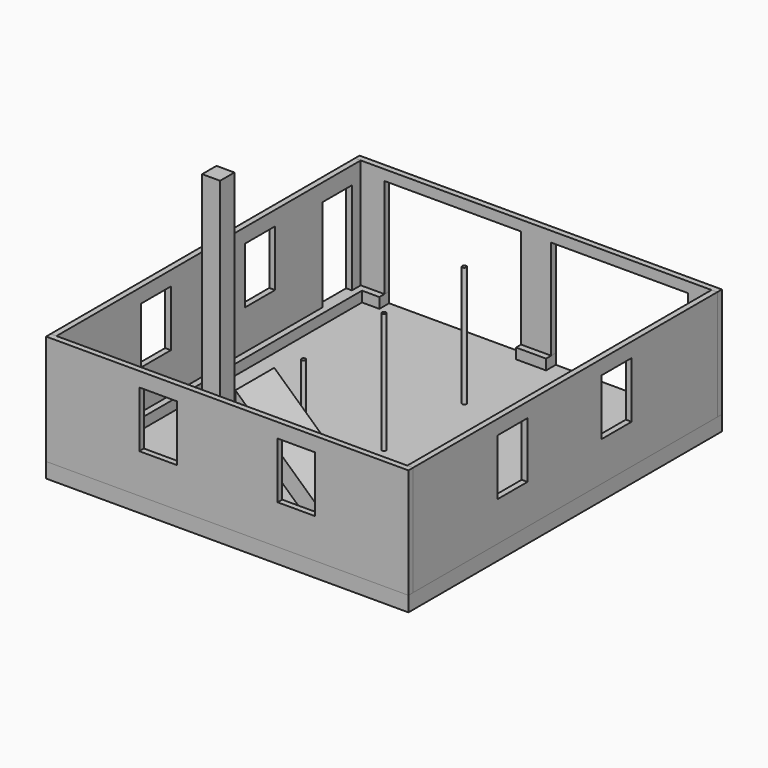
from build123d import *

# Parameters (mm, degrees)
F0_W      = 7950.2
F0_H      = 8597.9
F1_DEPTH  = 101.6
F2_W      = 660.4
F2_H      = 266.7
F3_DEPTH  = 228.6
F5_DEPTH  = 127
F6_W      = 7950.2
F6_H      = 2413
F6_W_2    = 825.5
F6_H_2    = 1231.9
F7_DEPTH  = 127
F8_W      = 825.5
F8_H      = 1231.9
F9_DEPTH  = 127
F10_W     = 8343.9
F10_H     = 2413
F11_DEPTH = 127
F12_DEPTH = 7950.2
F13_W     = 393.7
F13_H     = 393.7
F14_DEPTH = 6705.6
F15_W     = 1447.8
F15_H     = 1409.7
F16_DEPTH = 355.6
F17_W     = 1587.5
F17_H     = 279.4
F18_DEPTH = 177.8
F20_DEPTH = 1066.8
F21_R     = 44.45
F22_DEPTH = 2641.6


# Not quite as in the source:
# - a feature names something its author has since deleted; it is built from what else it names


with BuildPart() as f1:
    # F0 (on Top) → F1 (new body)
    with BuildSketch(Plane.XY):
        Rectangle(F0_W, F0_H)
    extrude(amount=-F1_DEPTH)

    # F2 (on face) → F3 (join)
    with BuildSketch(Plane.XY):
        Polygon((-3327.4, 4032.25), (-3327.4, 4298.95), (-3975.1, 4298.95), (-3975.1, -4298.95), (3975.1, -4298.95), (3975.1, 4298.95), (3327.4, 4298.95), (3327.4, 4032.25), (3708.4, 4032.25), (3708.4, -4032.25), (-3708.4, -4032.25), (-3708.4, 4032.25), align=None)
        with Locations((0, 4165.6)):
            Rectangle(F2_W, F2_H)
    extrude(amount=F3_DEPTH)

    # F21 (on face) → F22 (join, through all)
    with BuildSketch(Plane.XY):
        with Locations((0, 2203.45)):
            Circle(F21_R)
        Circle(F21_R)
        with Locations((0, -2203.45)):
            Circle(F21_R)
    extrude(amount=F22_DEPTH)


with BuildPart() as f5:
    # F4 (on face) → F5 (new body)
    with BuildSketch(Plane(origin=(0, 4298.95, 0), x_dir=(-1, 0, 0), z_dir=(0, 1, 0))):
        Polygon((-3975.1, 2641.6), (-3975.1, 228.6), (-3327.4, 228.6), (-3327.4, 2413), (-330.2, 2413), (-330.2, 228.6), (330.2, 228.6), (330.2, 2413), (3327.4, 2413), (3327.4, 228.6), (3975.1, 228.6), (3975.1, 2641.6), align=None)
    extrude(amount=-F5_DEPTH)


with BuildPart() as f7:
    # F6 (on face) → F7 (new body)
    with BuildSketch(Plane.XZ.offset(4298.95)):
        with Locations((0, 1435.1)):
            Rectangle(F6_W, F6_H)
        with Locations((-1517.65, 1708.15)):
            Rectangle(F6_W_2, F6_H_2, mode=Mode.SUBTRACT)
        with Locations((1517.65, 1708.15)):
            Rectangle(F6_W_2, F6_H_2, mode=Mode.SUBTRACT)
    extrude(amount=-F7_DEPTH)


with BuildPart() as f9:
    # F8 (on face) → F9 (new body)
    with BuildSketch(Plane(origin=(-3975.1, 0, 0), x_dir=(0, -1, 0), z_dir=(-1, 0, 0))):
        Polygon((4171.95, 2641.6), (-4171.95, 2641.6), (-4171.95, 228.6), (-3930.65, 228.6), (-3930.65, 2260.6), (-3117.85, 2260.6), (-3117.85, 228.6), (4171.95, 228.6), align=None)
        with Locations((-1409.7, 1708.15)):
            Rectangle(F8_W, F8_H, mode=Mode.SUBTRACT)
        with Locations((1447.8, 1708.15)):
            Rectangle(F8_W, F8_H, mode=Mode.SUBTRACT)
    extrude(amount=-F9_DEPTH)


with BuildPart() as f11:
    # F10 (on face) → F11 (new body)
    with BuildSketch(Plane.YZ.offset(3975.1)):
        with Locations((0, 1435.1)):
            Rectangle(F10_W, F10_H)
    extrude(amount=-F11_DEPTH)

    # F8 (on face) → F12 (cut, through all)
    with BuildSketch(Plane(origin=(-3975.1, 0, 0), x_dir=(0, -1, 0), z_dir=(-1, 0, 0))):
        with Locations((-1409.7, 1708.15)):
            Rectangle(F8_W, F8_H)
        with Locations((1447.8, 1708.15)):
            Rectangle(F8_W, F8_H)
    extrude(amount=-F12_DEPTH, mode=Mode.SUBTRACT)


with BuildPart() as f14:
    # F13 (on face) → F14 (new body)
    with BuildSketch(Plane.XY):
        with Locations((-577.85, -3822.7)):
            Rectangle(F13_W, F13_H)
    extrude(amount=F14_DEPTH)


with BuildPart() as f16:
    # F15 (on face) → F16 (new body)
    with BuildSketch(Plane.XY):
        with Locations((2984.5, -3327.4)):
            Rectangle(F15_W, F15_H)
        Polygon((2260.6, -4171.95), (3848.1, -4171.95), (3848.1, -2622.55), (3708.4, -2622.55), (3708.4, -4032.25), (2260.6, -4032.25), align=None)
    extrude(amount=F16_DEPTH)

    # F17 (on face) → F18 (cut)
    with BuildSketch(Plane.XY.offset(355.6)):
        with Locations((3054.35, -2762.25)):
            Rectangle(F17_W, F17_H)
    extrude(amount=-F18_DEPTH, mode=Mode.SUBTRACT)

    # F19 (on face) → F20 (join)
    with BuildSketch(Plane(origin=(0, -4171.95, 0), x_dir=(-1, 0, 0), z_dir=(0, 1, 0))):
        Polygon((-2628.9, 355.6), (-2260.6, 355.6), (-76.2, 2355.2497512438), (-76.2, 2870.2), (-2628.9, 533.4), align=None)
    extrude(amount=F20_DEPTH)


solid = Compound([f1.part, f5.part, f7.part, f9.part, f11.part, f14.part, f16.part])
